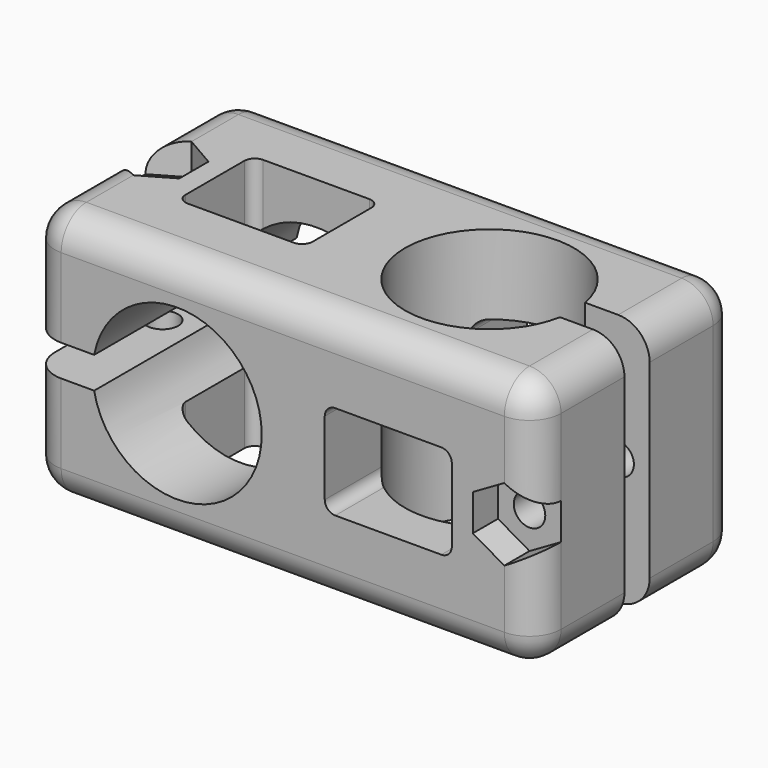
from build123d import *

# Parameters (mm, degrees)
F0_W          = 48.2
F0_H          = 24.1
F0_W_2        = 12.1
F0_H_2        = 9
F0_R          = 8.05
F1_DEPTH      = 12.05
F2_R          = 8.05
F2_W          = 12.1
F2_H          = 9
F3_DEPTH      = 25
F4_W          = 20.2092044055
F4_H          = 3
F5_DEPTH      = 25
F6_W          = 15.0541103601
F6_H          = 3
F7_DEPTH      = 24.101
F9_DEPTH      = 3
F10_R         = 1.5
F11_DEPTH     = 21.101
F12_R         = 2.5
F13_DEPTH     = 3
F14_R         = 1
F16_DEPTH     = 3
F17_R         = 1.5
F18_DEPTH     = 21.1010001
F19_R         = 2.5
F20_DEPTH     = 3
F21_T1_DEPTH  = 18.1
F21_T3_DEPTH  = 42.2
F21_T5_DEPTH  = 15.05
F21_T7_DEPTH  = 15.05
F21_T9_DEPTH  = 14.8179491924
F21_T11_DEPTH = 14.8179491924
F21_T13_DEPTH = 18.1
F21_T15_DEPTH = 14.8179491924
F21_T17_DEPTH = 14.8179491924
F21_T19_DEPTH = 15.05
F21_T21_DEPTH = 15.05
F21_S25_W     = 3
F21_S25_H     = 3
F21_T26_DEPTH = 3
F21_S31_W     = 3
F21_S31_H     = 3
F21_T32_DEPTH = 3
F21_S37_W     = 3
F21_S37_H     = 3
F21_T38_DEPTH = 3
F21_S43_W     = 3
F21_S43_H     = 3
F21_T44_DEPTH = 3
F21_S49_W     = 3
F21_S49_H     = 3
F21_T50_DEPTH = 3
F21_S55_W     = 3
F21_S55_H     = 3
F21_T56_DEPTH = 3
F21_S61_W     = 3
F21_S61_H     = 3
F21_T62_DEPTH = 3
F21_S67_W     = 3
F21_S67_H     = 3
F21_T68_DEPTH = 3


# Not quite as in the source:
# - a fillet or chamfer that OpenCascade refuses, or shapes differently, is made with other operations: its cross-section is extruded or revolved along the edge and cut away or added


with BuildPart() as f1:
    # F0 (on Top) → F1 (new body, symmetric)
    with BuildSketch(Plane.XY):
        Rectangle(F0_W, F0_H)
        with Locations((-10.05, 0)):
            Rectangle(F0_W_2, F0_H_2, mode=Mode.SUBTRACT)
        with Locations((10.05, 0)):
            Circle(F0_R, mode=Mode.SUBTRACT)
    extrude(amount=F1_DEPTH, both=True)

    # F2 (on face) → F3 (cut)
    with BuildSketch(Plane.XZ.offset(12.05)):
        with Locations((-10.05, 0)):
            Circle(F2_R)
        with Locations((10.05, 0)):
            Rectangle(F2_W, F2_H)
    extrude(amount=-F3_DEPTH, mode=Mode.SUBTRACT)

    # F4 (on face) → F5 (cut)
    with BuildSketch(Plane(origin=(0, 12.05, 0), x_dir=(-1, 0, 0), z_dir=(0, 1, 0))):
        with Locations((26.3627953827, 0)):
            Rectangle(F4_W, F4_H)
    extrude(amount=-F5_DEPTH, mode=Mode.SUBTRACT)

    # F6 (on face) → F7 (cut, through all)
    with BuildSketch(Plane(origin=(0, 0, -12.05), x_dir=(1, 0, 0), z_dir=(0, 0, -1))):
        with Locations((24.1, 0)):
            Rectangle(F6_W, F6_H)
    extrude(amount=-F7_DEPTH, mode=Mode.SUBTRACT)

    # F8 (on face) → F9 (cut)
    with BuildSketch(Plane.XZ.offset(12.05)):
        Polygon((21.1, 3.4641016151), (18.1, 1.7320508076), (18.1, -1.7320508076), (21.1, -3.4641016151), (24.1, -1.7320508076), (24.1, 1.7320508076), align=None)
    extrude(amount=-F9_DEPTH, mode=Mode.SUBTRACT)

    # F10 (on face) → F11 (cut, through all)
    with BuildSketch(Plane.XZ.offset(9.05)):
        with Locations((21.1, 0)):
            Circle(F10_R)
    extrude(amount=-F11_DEPTH, mode=Mode.SUBTRACT)

    # F12 (on face) → F13 (cut)
    with BuildSketch(Plane(origin=(0, 12.05, 0), x_dir=(-1, 0, 0), z_dir=(0, 1, 0))):
        with Locations((-21.1, 0)):
            Circle(F12_R)
    extrude(amount=-F13_DEPTH, mode=Mode.SUBTRACT)

    # F14
    f14_edges = [f1.edges().sort_by_distance(p)[0] for p in [
        (16.1, -8.680184, 4.5),
        (16.1, -8.680184, -4.5),
        (4, -8.680184, 4.5),
        (4, -8.680184, -4.5),
        (-4, -4.5, 8.680184),
        (-4, 4.5, 8.680184),
        (-16.1, -4.5, 8.680184),
        (-16.1, 4.5, 8.680184),
        (-4, 4.5, -8.680184),
        (-16.1, 4.5, -8.680184),
        (-16.1, -4.5, -8.680184),
        (-4, -4.5, -8.680184),
        (4, 8.680184, 4.5),
        (16.1, 8.680184, 4.5),
        (16.1, 8.680184, -4.5),
        (4, 8.680184, -4.5),
    ]]
    fillet(f14_edges, radius=F14_R)

    # F15 (on face) → F16 (cut)
    with BuildSketch(Plane.XY.offset(12.05)):
        Polygon((-21.1, 3.4641016151), (-24.1, 1.7320508076), (-24.1, -1.7320508076), (-21.1, -3.4641016151), (-18.1, -1.7320508076), (-18.1, 1.7320508076), align=None)
    extrude(amount=-F16_DEPTH, mode=Mode.SUBTRACT)

    # F17 (on face) → F18 (cut, through all)
    with BuildSketch(Plane.XY.offset(9.05)):
        with Locations((-21.1, 0)):
            Circle(F17_R)
    extrude(amount=-F18_DEPTH, mode=Mode.SUBTRACT)

    # F19 (on face) → F20 (cut)
    with BuildSketch(Plane(origin=(0, 0, -12.05), x_dir=(1, 0, 0), z_dir=(0, 0, -1))):
        with Locations((-21.1, 0)):
            Circle(F19_R)
    extrude(amount=-F20_DEPTH, mode=Mode.SUBTRACT)

    # F21: fillet of radius 3 on 18 edges, made by hand

    # F21_s2 → F21_t1 (cut)
    with BuildSketch(Plane.XZ.offset(-9.05)):
        with BuildLine():
            ThreePointArc((-21.1, -12.05), (-23.2213203436, -11.1713203436), (-24.1, -9.05))
            Line((-24.1, -9.05), (-24.1, -12.05))
            Line((-24.1, -12.05), (-21.1, -12.05))
        make_face()
    extrude(amount=F21_T1_DEPTH, mode=Mode.SUBTRACT)

    # F21_s4 → F21_t3 (cut)
    with BuildSketch(Plane.YZ.offset(-21.1)):
        with BuildLine():
            ThreePointArc((-9.05, -12.05), (-11.1713203436, -11.1713203436), (-12.05, -9.05))
            Line((-12.05, -9.05), (-12.05, -12.05))
            Line((-12.05, -12.05), (-9.05, -12.05))
        make_face()
        with BuildLine():
            ThreePointArc((12.05, -9.05), (11.1713203436, -11.1713203436), (9.05, -12.05))
            Line((9.05, -12.05), (12.05, -12.05))
            Line((12.05, -12.05), (12.05, -9.05))
        make_face()
        with BuildLine():
            ThreePointArc((12.05, 9.05), (11.1713203436, 11.1713203436), (9.05, 12.05))
            Line((9.05, 12.05), (12.05, 12.05))
            Line((12.05, 12.05), (12.05, 9.05))
        make_face()
        with BuildLine():
            ThreePointArc((-9.05, 12.05), (-11.1713203436, 11.1713203436), (-12.05, 9.05))
            Line((-12.05, 9.05), (-12.05, 12.05))
            Line((-12.05, 12.05), (-9.05, 12.05))
        make_face()
    extrude(amount=F21_T3_DEPTH, mode=Mode.SUBTRACT)

    # F21_s6 → F21_t5 (cut)
    with BuildSketch(Plane.XZ.offset(-9.05)):
        with BuildLine():
            ThreePointArc((24.1, -9.05), (23.2213203436, -11.1713203436), (21.1, -12.05))
            Line((21.1, -12.05), (24.1, -12.05))
            Line((24.1, -12.05), (24.1, -9.05))
        make_face()
        with BuildLine():
            ThreePointArc((24.1, 9.05), (23.2213203436, 11.1713203436), (21.1, 12.05))
            Line((21.1, 12.05), (24.1, 12.05))
            Line((24.1, 12.05), (24.1, 9.05))
        make_face()
    extrude(amount=F21_T5_DEPTH, mode=Mode.SUBTRACT)

    # F21_s8 → F21_t7 (cut)
    with BuildSketch(Plane.XZ.offset(-6)):
        with BuildLine():
            ThreePointArc((21.1, -12.05), (23.2213203436, -11.1713203436), (24.1, -9.05))
            Line((24.1, -9.05), (24.1, -12.05))
            Line((24.1, -12.05), (21.1, -12.05))
        make_face()
        with BuildLine():
            ThreePointArc((21.1, 12.05), (23.2213203436, 11.1713203436), (24.1, 9.05))
            Line((24.1, 9.05), (24.1, 12.05))
            Line((24.1, 12.05), (21.1, 12.05))
        make_face()
    extrude(amount=F21_T7_DEPTH, mode=Mode.SUBTRACT)

    # F21_s10 → F21_t9 (cut)
    with BuildSketch(Plane.XY.offset(-9.05)):
        with BuildLine():
            ThreePointArc((24.1, -9.05), (23.2213203436, -11.1713203436), (21.1, -12.05))
            Line((21.1, -12.05), (24.1, -12.05))
            Line((24.1, -12.05), (24.1, -9.05))
        make_face()
    extrude(amount=F21_T9_DEPTH, mode=Mode.SUBTRACT)

    # F21_s12 → F21_t11 (cut)
    with BuildSketch(Plane.XY.offset(-5.7679491924)):
        with BuildLine():
            ThreePointArc((24.1, -9.05), (23.2213203436, -11.1713203436), (21.1, -12.05))
            Line((21.1, -12.05), (24.1, -12.05))
            Line((24.1, -12.05), (24.1, -9.05))
        make_face()
    extrude(amount=F21_T11_DEPTH, mode=Mode.SUBTRACT)

    # F21_s14 → F21_t13 (cut)
    with BuildSketch(Plane.XY.offset(-9.05)):
        with BuildLine():
            ThreePointArc((21.1, 12.05), (23.2213203436, 11.1713203436), (24.1, 9.05))
            Line((24.1, 9.05), (24.1, 12.05))
            Line((24.1, 12.05), (21.1, 12.05))
        make_face()
    extrude(amount=F21_T13_DEPTH, mode=Mode.SUBTRACT)

    # F21_s16 → F21_t15 (cut)
    with BuildSketch(Plane.XZ.offset(-5.7679491924)):
        with BuildLine():
            ThreePointArc((-21.1, 12.05), (-23.2213203436, 11.1713203436), (-24.1, 9.05))
            Line((-24.1, 9.05), (-24.1, 12.05))
            Line((-24.1, 12.05), (-21.1, 12.05))
        make_face()
    extrude(amount=F21_T15_DEPTH, mode=Mode.SUBTRACT)

    # F21_s18 → F21_t17 (cut)
    with BuildSketch(Plane.XZ.offset(-9.05)):
        with BuildLine():
            ThreePointArc((-21.1, 12.05), (-23.2213203436, 11.1713203436), (-24.1, 9.05))
            Line((-24.1, 9.05), (-24.1, 12.05))
            Line((-24.1, 12.05), (-21.1, 12.05))
        make_face()
    extrude(amount=F21_T17_DEPTH, mode=Mode.SUBTRACT)

    # F21_s20 → F21_t19 (cut)
    with BuildSketch(Plane.XY.offset(-6)):
        with BuildLine():
            ThreePointArc((-24.1, -9.05), (-23.2213203436, -11.1713203436), (-21.1, -12.05))
            Line((-21.1, -12.05), (-24.1, -12.05))
            Line((-24.1, -12.05), (-24.1, -9.05))
        make_face()
        with BuildLine():
            ThreePointArc((-21.1, 12.05), (-23.2213203436, 11.1713203436), (-24.1, 9.05))
            Line((-24.1, 9.05), (-24.1, 12.05))
            Line((-24.1, 12.05), (-21.1, 12.05))
        make_face()
    extrude(amount=F21_T19_DEPTH, mode=Mode.SUBTRACT)

    # F21_s22 → F21_t21 (cut)
    with BuildSketch(Plane.XY.offset(-9.05)):
        with BuildLine():
            ThreePointArc((-24.1, -9.05), (-23.2213203436, -11.1713203436), (-21.1, -12.05))
            Line((-21.1, -12.05), (-24.1, -12.05))
            Line((-24.1, -12.05), (-24.1, -9.05))
        make_face()
        with BuildLine():
            ThreePointArc((-21.1, 12.05), (-23.2213203436, 11.1713203436), (-24.1, 9.05))
            Line((-24.1, 9.05), (-24.1, 12.05))
            Line((-24.1, 12.05), (-21.1, 12.05))
        make_face()
    extrude(amount=F21_T21_DEPTH, mode=Mode.SUBTRACT)


with BuildPart() as f21_tool24:
    # F21_s25 → F21_t26 (new body)
    with BuildSketch(Plane.XZ.offset(-9.05)):
        with Locations((-22.6, -10.55)):
            Rectangle(F21_S25_W, F21_S25_H)
    extrude(amount=-F21_T26_DEPTH)

    # F21_s27 → F21_t28 (revolve, cut)
    with BuildSketch(Plane(origin=(-21.1, 9.05, -9.05), x_dir=(0.7071067812, 0, 0.7071067812), z_dir=(-0.7071067812, 0, 0.7071067812))):
        with BuildLine():
            ThreePointArc((0, -3), (3, 0), (0, 3))
            Line((0, 3), (0, -3))
        make_face()
    revolve(axis=Axis((-21.1, 9.05, -9.05), (0, 1, 0)), mode=Mode.SUBTRACT)


with BuildPart() as f1_1:
    add(f1.part)

    # F21_t23: cut F21_tool24
    add(f21_tool24.part, mode=Mode.SUBTRACT)


with BuildPart() as f21_tool30:
    # F21_s31 → F21_t32 (new body)
    with BuildSketch(Plane.XY.offset(-9.05)):
        with Locations((-22.6, -10.55)):
            Rectangle(F21_S31_W, F21_S31_H)
    extrude(amount=-F21_T32_DEPTH)

    # F21_s33 → F21_t34 (revolve, cut)
    with BuildSketch(Plane(origin=(-21.1, -9.05, -9.05), x_dir=(0.7071067812, 0.7071067812, 0), z_dir=(-0.7071067812, 0.7071067812, 0))):
        with BuildLine():
            ThreePointArc((0, -3), (3, 0), (0, 3))
            Line((0, 3), (0, -3))
        make_face()
    revolve(axis=Axis((-21.1, -9.05, -9.05), (0, 0, -1)), mode=Mode.SUBTRACT)


with BuildPart() as f1_2:
    add(f1_1.part)

    # F21_t29: cut F21_tool30
    add(f21_tool30.part, mode=Mode.SUBTRACT)


with BuildPart() as f21_tool36:
    # F21_s37 → F21_t38 (new body)
    with BuildSketch(Plane.XY.offset(-9.05)):
        with Locations((22.6, -10.55)):
            Rectangle(F21_S37_W, F21_S37_H)
    extrude(amount=-F21_T38_DEPTH)

    # F21_s39 → F21_t40 (revolve, cut)
    with BuildSketch(Plane(origin=(21.1, -9.05, -9.05), x_dir=(-0.7071067812, 0.7071067812, 0), z_dir=(-0.7071067812, -0.7071067812, 0))):
        with BuildLine():
            ThreePointArc((0, -3), (3, 0), (0, 3))
            Line((0, 3), (0, -3))
        make_face()
    revolve(axis=Axis((21.1, -9.05, -9.05), (0, 0, -1)), mode=Mode.SUBTRACT)


with BuildPart() as f1_3:
    add(f1_2.part)

    # F21_t35: cut F21_tool36
    add(f21_tool36.part, mode=Mode.SUBTRACT)


with BuildPart() as f21_tool42:
    # F21_s43 → F21_t44 (new body)
    with BuildSketch(Plane.XZ.offset(-9.05)):
        with Locations((22.6, -10.55)):
            Rectangle(F21_S43_W, F21_S43_H)
    extrude(amount=-F21_T44_DEPTH)

    # F21_s45 → F21_t46 (revolve, cut)
    with BuildSketch(Plane(origin=(21.1, 9.05, -9.05), x_dir=(-0.7071067812, 0, 0.7071067812), z_dir=(-0.7071067812, 0, -0.7071067812))):
        with BuildLine():
            ThreePointArc((0, -3), (3, 0), (0, 3))
            Line((0, 3), (0, -3))
        make_face()
    revolve(axis=Axis((21.1, 9.05, -9.05), (0, 1, 0)), mode=Mode.SUBTRACT)


with BuildPart() as f1_4:
    add(f1_3.part)

    # F21_t41: cut F21_tool42
    add(f21_tool42.part, mode=Mode.SUBTRACT)


with BuildPart() as f21_tool48:
    # F21_s49 → F21_t50 (new body)
    with BuildSketch(Plane.XY.offset(9.05)):
        with Locations((22.6, -10.55)):
            Rectangle(F21_S49_W, F21_S49_H)
    extrude(amount=F21_T50_DEPTH)

    # F21_s51 → F21_t52 (revolve, cut)
    with BuildSketch(Plane(origin=(21.1, -9.05, 9.05), x_dir=(-0.7071067812, 0.7071067812, 0), z_dir=(0.7071067812, 0.7071067812, 0))):
        with BuildLine():
            ThreePointArc((0, -3), (3, 0), (0, 3))
            Line((0, 3), (0, -3))
        make_face()
    revolve(axis=Axis((21.1, -9.05, 9.05), (0, 0, 1)), mode=Mode.SUBTRACT)


with BuildPart() as f1_5:
    add(f1_4.part)

    # F21_t47: cut F21_tool48
    add(f21_tool48.part, mode=Mode.SUBTRACT)


with BuildPart() as f21_tool54:
    # F21_s55 → F21_t56 (new body)
    with BuildSketch(Plane.XZ.offset(-9.05)):
        with Locations((22.6, 10.55)):
            Rectangle(F21_S55_W, F21_S55_H)
    extrude(amount=-F21_T56_DEPTH)

    # F21_s57 → F21_t58 (revolve, cut)
    with BuildSketch(Plane(origin=(21.1, 9.05, 9.05), x_dir=(-0.7071067812, 0, -0.7071067812), z_dir=(0.7071067812, 0, -0.7071067812))):
        with BuildLine():
            ThreePointArc((0, -3), (3, 0), (0, 3))
            Line((0, 3), (0, -3))
        make_face()
    revolve(axis=Axis((21.1, 9.05, 9.05), (0, 1, 0)), mode=Mode.SUBTRACT)


with BuildPart() as f1_6:
    add(f1_5.part)

    # F21_t53: cut F21_tool54
    add(f21_tool54.part, mode=Mode.SUBTRACT)


with BuildPart() as f21_tool60:
    # F21_s61 → F21_t62 (new body)
    with BuildSketch(Plane.XZ.offset(-9.05)):
        with Locations((-22.6, 10.55)):
            Rectangle(F21_S61_W, F21_S61_H)
    extrude(amount=-F21_T62_DEPTH)

    # F21_s63 → F21_t64 (revolve, cut)
    with BuildSketch(Plane(origin=(-21.1, 9.05, 9.05), x_dir=(0.7071067812, 0, -0.7071067812), z_dir=(0.7071067812, 0, 0.7071067812))):
        with BuildLine():
            ThreePointArc((0, -3), (3, 0), (0, 3))
            Line((0, 3), (0, -3))
        make_face()
    revolve(axis=Axis((-21.1, 9.05, 9.05), (0, 1, 0)), mode=Mode.SUBTRACT)


with BuildPart() as f1_7:
    add(f1_6.part)

    # F21_t59: cut F21_tool60
    add(f21_tool60.part, mode=Mode.SUBTRACT)


with BuildPart() as f21_tool66:
    # F21_s67 → F21_t68 (new body)
    with BuildSketch(Plane.XY.offset(9.05)):
        with Locations((-22.6, -10.55)):
            Rectangle(F21_S67_W, F21_S67_H)
    extrude(amount=F21_T68_DEPTH)

    # F21_s69 → F21_t70 (revolve, cut)
    with BuildSketch(Plane(origin=(-21.1, -9.05, 9.05), x_dir=(0.7071067812, 0.7071067812, 0), z_dir=(0.7071067812, -0.7071067812, 0))):
        with BuildLine():
            ThreePointArc((0, -3), (3, 0), (0, 3))
            Line((0, 3), (0, -3))
        make_face()
    revolve(axis=Axis((-21.1, -9.05, 9.05), (0, 0, 1)), mode=Mode.SUBTRACT)


with BuildPart() as f1_8:
    add(f1_7.part)

    # F21_t65: cut F21_tool66
    add(f21_tool66.part, mode=Mode.SUBTRACT)


solid = f1_8.part
